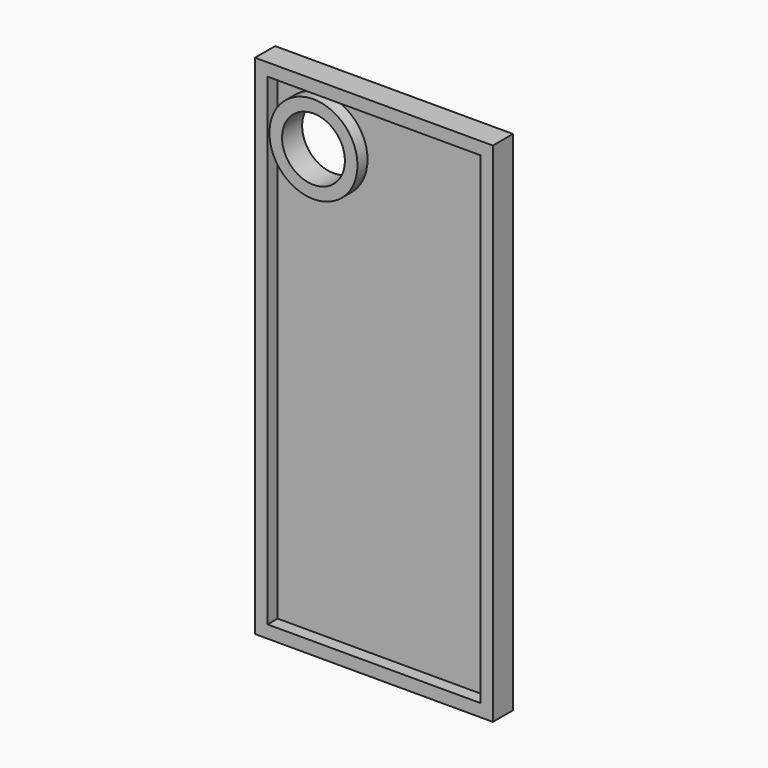
from build123d import *

# Parameters (mm, degrees)
F0_W         = 48.0267032981
F0_H         = 102.470766753
F1_DEPTH     = 5.08
F3_D         = 12.7
F4_T         = -2.54
F5_TEXT_SIZE = 17.2727916696
F6_DEPTH     = 1.04659
F7_TEXT_SIZE = 15.9799263606
F8_DEPTH     = 0.762


# Not quite as in the source:
# - Text() gives the source's letters only with a copy of the font that has no kerning and outlines rounded to 1/6400 em; it was checked with that copy


with BuildPart() as f1:
    # F0 (on Front) → F1 (new body)
    with BuildSketch(Plane.XZ):
        with Locations((-0.93155168, -1.8631052226)):
            Rectangle(F0_W, F0_H)
    extrude(amount=F1_DEPTH)

    # F3 (through all)
    with Locations(Plane(origin=(0, 0, 0), x_dir=(-1, 0, 0), z_dir=(0, 1, 0))):
        with Locations((13.1452409551, 36.9515791535)):
            Hole(F3_D / 2)

    # F4
    f4_openings = [f1.faces().sort_by_distance(p)[0] for p in [
        (-0.608861, -5.08, -2.888606),
    ]]
    offset(amount=F4_T, openings=f4_openings)

    # F5 (on face) → F6 (join)
    with BuildSketch(Plane(origin=(0, 0, 0), x_dir=(-1, 0, 0), z_dir=(0, 1, 0))):
        with Locations((-18.4762504854, 0)):
            Text('LIVE!', F5_TEXT_SIZE, font='Open Sans', text_align=(TextAlign.LEFT, TextAlign.BOTTOM))
    extrude(amount=F6_DEPTH)

    # F7 (on face) → F8 (join)
    with BuildSketch(Plane(origin=(0, 0, 0), x_dir=(-1, 0, 0), z_dir=(0, 1, 0))):
        with Locations((-20.8410862833, -25.5312994123)):
            Text('HOPE!', F7_TEXT_SIZE, font='Open Sans', text_align=(TextAlign.LEFT, TextAlign.BOTTOM))
    extrude(amount=F8_DEPTH)


solid = f1.part
